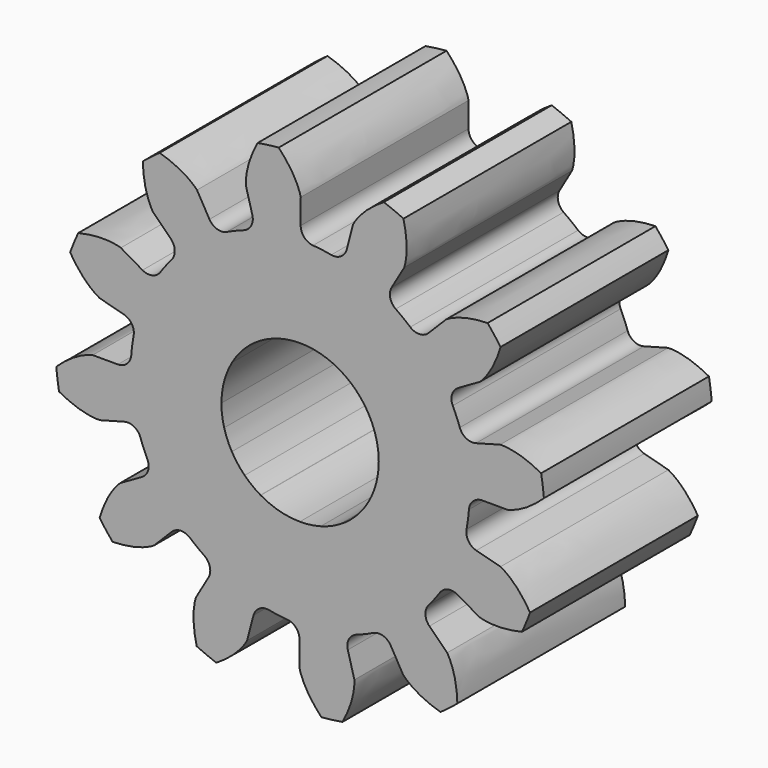
from build123d import *

# Parameters (mm, degrees)
F3_DEPTH        = 3.175
F3_COPIES_COUNT = 12
F4_R            = 0.2032


# Not quite as in the source:
# - a feature of the source that left no trace in its solid (it failed there, or was rolled back) is left out
# - a pattern or mirror of a feature is missing from the dataset's text; its kind, count and spacing are read off the source's solid


with BuildPart() as f3:
    # F2 (on Front) → F3 (new body)
    with BuildSketch(Plane.XZ):
        with BuildLine():
            add(Edge.make_bspline(
                [(-0.3234027057, 3.6900218677), (-0.2333809861, 3.5889719035), (-0.2583485947, 3.6207458775), (-0.1530135495, 3.4866956752), (-0.1027187311, 3.4060434713), (-0.0558207338, 3.3194897709), (-0.0262314445, 3.2548922221), (0.0023217415, 3.1704242627), (-0.0031871923, 3.1867211618), (0.01005916, 3.1380066115)],
                knots=[0, 0, 0, 0, 0.1743394157, 0.3394849194, 0.4948101285, 0.6395714738, 0.772859937, 0.8935199848, 1, 1, 1, 1], degree=3))
            ThreePointArc((-0.3234027057, 3.6900218677), (-0.4834907703, 3.6724770073), (-0.6426649105, 3.6479902011))
            add(Edge.make_bspline(
                [(-0.6426649105, 3.6479902011), (-0.7034655592, 3.5270840954), (-0.6875724108, 3.5642374901), (-0.754623506, 3.4074922218), (-0.7823302436, 3.3165709183), (-0.8052284843, 3.2208283688), (-0.8170904672, 3.1507736566), (-0.8228088103, 3.0617937647), (-0.8217055368, 3.0789611774), (-0.8218922772, 3.028478127)],
                knots=[0, 0, 0, 0, 0.1743394157, 0.3394849194, 0.4948101285, 0.6395714738, 0.772859937, 0.8935199848, 1, 1, 1, 1], degree=3))
            Line((-0.8218922772, 3.028478127), (-0.6712213506, 2.4732914946))
            ThreePointArc((-0.6712213506, 2.4732914946), (-0.334506543, 2.5408294495), (0.0082150948, 2.5627409996))
            Line((0.0082150948, 2.5627409996), (0.01005916, 3.1380066115))
        make_face()
        with BuildLine():
            Line((0.003816635, 1.1906188827), (0.0082150948, 2.5627409996))
            ThreePointArc((0.0082150948, 2.5627409996), (-0.334506543, 2.5408294495), (-0.6712213506, 2.4732914946))
            Line((-0.6712213506, 2.4732914946), (-0.3118414286, 1.1490617103))
            ThreePointArc((-0.3118414286, 1.1490617103), (-0.1554077476, 1.1804390381), (0.003816635, 1.1906188827))
        make_face()
        with BuildLine():
            ThreePointArc((2.5627541667, 0), (1.8150430005, 1.8092340438), (0.0082150948, 2.5627409996))
            Line((0.0082150948, 2.5627409996), (0.003816635, 1.1906188827))
            ThreePointArc((0.003816635, 1.1906188827), (0.8432473159, 0.840548544), (1.190625, 0))
            ThreePointArc((1.190625, 0), (-0.7232916734, -0.9457468191), (-0.3118414286, 1.1490617103))
            Line((-0.3118414286, 1.1490617103), (-0.6712213506, 2.4732914946))
            ThreePointArc((-0.6712213506, 2.4732914946), (-1.5568451442, -2.0356674866), (2.5627541667, 0))
        make_face()
    extrude(amount=F3_DEPTH)

    # F3_copies: F3 ×12 about axis
    f3_copies_axis = Axis((0, 0, 0), (0, 1, 0))


with BuildPart() as f3_1:
    add(f3.part)
    for i in range(1, F3_COPIES_COUNT):
        add(f3.part.rotate(f3_copies_axis, i * 360 / F3_COPIES_COUNT))

    # F4
    f4_edges = [f3_1.edges().sort_by_distance(p)[0] for p in [
        (2.562741, -1.5875, -0.008215),
        (-0.671221, -1.5875, 2.473291),
        (-1.274256, -1.5875, 2.223506),
        (-1.81794, -1.5875, 1.806323),
        (-2.215291, -1.5875, 1.288485),
        (-2.477544, -1.5875, 0.655351),
        (-2.562741, -1.5875, 0.008215),
        (-2.473291, -1.5875, -0.671221),
        (-2.223506, -1.5875, -1.274256),
        (-1.806323, -1.5875, -1.81794),
        (-1.288485, -1.5875, -2.215291),
        (-0.655351, -1.5875, -2.477544),
        (-0.008215, -1.5875, -2.562741),
        (0.671221, -1.5875, -2.473291),
        (1.274256, -1.5875, -2.223506),
        (1.81794, -1.5875, -1.806323),
        (2.215291, -1.5875, -1.288485),
        (2.477544, -1.5875, -0.655351),
        (2.473291, -1.5875, 0.671221),
        (2.223506, -1.5875, 1.274256),
        (1.806323, -1.5875, 1.81794),
        (1.288485, -1.5875, 2.215291),
        (0.655351, -1.5875, 2.477544),
        (0.008215, -1.5875, 2.562741),
    ]]
    fillet(f4_edges, radius=F4_R)


solid = f3_1.part
